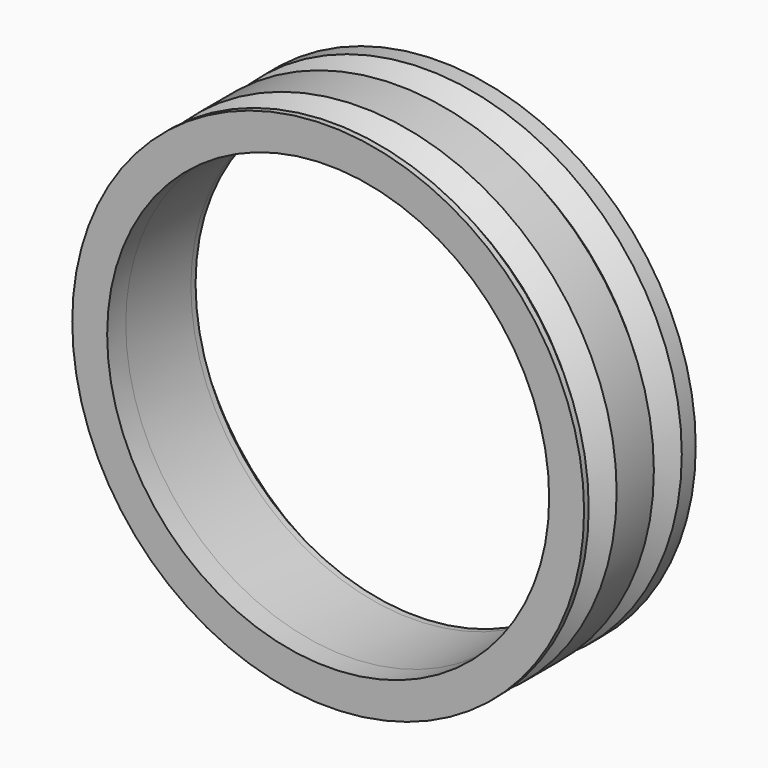
from build123d import *

# Parameters (mm, degrees)
F0_R     = 22
F0_R_2   = 19
F1_DEPTH = 7
F2_SIZE  = 1.5
F3_R     = 22
F3_R_2   = 19
F4_DEPTH = 3
F5_SIZE  = 1.49999
F6_SIZE  = 2.5
F7_SIZE  = 1.5
F8_R     = 22
F8_R_2   = 19
F9_DEPTH = 2
F10_SIZE = 1.49999


# Not quite as in the source:
# - a fillet or chamfer is up to 0.001 mm smaller than in the source, because OpenCascade refuses the exact size


with BuildPart() as f1:
    # F0 (on Front) → F1 (new body)
    with BuildSketch(Plane.XZ):
        Circle(F0_R)
        Circle(F0_R_2, mode=Mode.SUBTRACT)
    extrude(amount=F1_DEPTH)

    # F2
    f2_edges = [f1.edges().sort_by_distance(p)[0] for p in [
        (-22, 0, 0),
    ]]
    chamfer(f2_edges, length=F2_SIZE)

    # F3 (on face) → F4 (join)
    with BuildSketch(Plane(origin=(0, 0, 0), x_dir=(-1, 0, 0), z_dir=(0, 1, 0))):
        Circle(F3_R)
        Circle(F3_R_2, mode=Mode.SUBTRACT)
    extrude(amount=F4_DEPTH)

    # F5 (size 1.5 in the source; OpenCascade refuses exactly that, so slightly less here)
    f5_edges = [f1.edges().sort_by_distance(p)[0] for p in [
        (22, 0, 0),
    ]]
    chamfer(f5_edges, length=F5_SIZE)

    # F6
    f6_edges = [f1.edges().sort_by_distance(p)[0] for p in [
        (19, 3, 0),
    ]]
    chamfer(f6_edges, length=F6_SIZE)

    # F7
    f7_edges = [f1.edges().sort_by_distance(p)[0] for p in [
        (-22, -7, 0),
    ]]
    chamfer(f7_edges, length=F7_SIZE)

    # F8 (on face) → F9 (join)
    with BuildSketch(Plane.XZ.offset(7)):
        Circle(F8_R)
        Circle(F8_R_2, mode=Mode.SUBTRACT)
    extrude(amount=F9_DEPTH)

    # F10 (size 1.5 in the source; OpenCascade refuses exactly that, so slightly less here)
    f10_edges = [f1.edges().sort_by_distance(p)[0] for p in [
        (-22, -7, 0),
    ]]
    chamfer(f10_edges, length=F10_SIZE)


solid = f1.part
